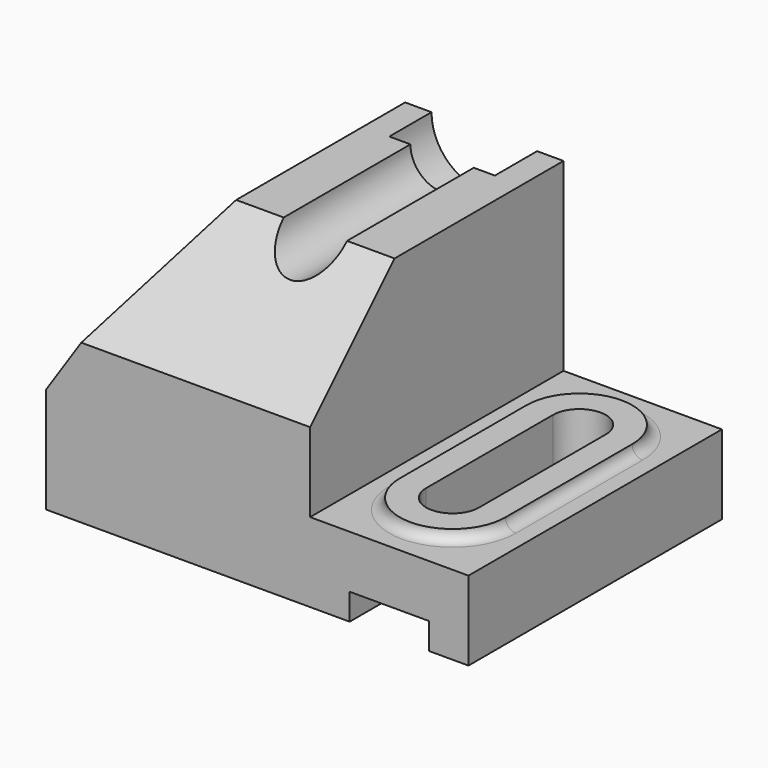
from build123d import *

# Parameters (mm, degrees)
F0_W         = 80
F0_H         = 60
F1_DEPTH     = 50
F2_W         = 30
F2_H         = 33
F3_DEPTH     = 60.001
F5_DEPTH     = 17.001
F6_W         = 30
F6_H         = 60
F7_DEPTH     = 2
F8_W         = 15
F8_H         = 5
F9_DEPTH     = 60.001
F10_R        = 1.99999
F12_DEPTH    = 60.001
F13_W        = 6
F13_H        = 48.9288835973
F15_W        = 4
F15_H        = 10
F17_T1_DEPTH = 132.8673195186


# Not quite as in the source:
# - a fillet or chamfer that OpenCascade refuses, or shapes differently, is made with other operations: its cross-section is extruded or revolved along the edge and cut away or added
# - a fillet or chamfer is up to 0.001 mm smaller than in the source, because OpenCascade refuses the exact size


with BuildPart() as f1:
    # F0 (on Top) → F1 (new body)
    with BuildSketch(Plane.XY):
        Rectangle(F0_W, F0_H)
    extrude(amount=F1_DEPTH)

    # F2 (on face) → F3 (cut, through all)
    with BuildSketch(Plane.XZ.offset(30)):
        with Locations((25, 33.5)):
            Rectangle(F2_W, F2_H)
    extrude(amount=-F3_DEPTH, mode=Mode.SUBTRACT)

    # F4 (on face) → F5 (cut, through all)
    with BuildSketch(Plane.XY.offset(17)):
        with BuildLine():
            ThreePointArc((20, -15), (25, -20), (30, -15))
            Line((30, -15), (30, 15))
            ThreePointArc((30, 15), (25, 20), (20, 15))
            Line((20, 15), (20, -15))
        make_face()
    extrude(amount=-F5_DEPTH, mode=Mode.SUBTRACT)

    # F6 (on face) → F7 (cut)
    with BuildSketch(Plane.XY.offset(17)):
        with Locations((25, 0)):
            Rectangle(F6_W, F6_H)
        with BuildLine():
            Line((35, 15), (35, -15))
            ThreePointArc((35, -15), (25, -25), (15, -15))
            Line((15, -15), (15, 15))
            ThreePointArc((15, 15), (25, 25), (35, 15))
        make_face(mode=Mode.SUBTRACT)
    extrude(amount=-F7_DEPTH, mode=Mode.SUBTRACT)

    # F8 (on face) → F9 (cut, through all)
    with BuildSketch(Plane.XZ.offset(30)):
        with Locations((25, 2.5)):
            Rectangle(F8_W, F8_H)
    extrude(amount=-F9_DEPTH, mode=Mode.SUBTRACT)

    # F10 (radius 2 in the source; OpenCascade refuses exactly that, so slightly less here)
    f10_edges = [f1.edges().sort_by_distance(p)[0] for p in [
        (35, 0, 15),
    ]]
    fillet(f10_edges, radius=F10_R)

    # F11 (on face) → F12 (cut, through all)
    with BuildSketch(Plane.XZ.offset(30)):
        Polygon((-40, 20), (-20, 50), (-40, 50), align=None)
    extrude(amount=-F12_DEPTH, mode=Mode.SUBTRACT)

    # F13 (on face) → F14 (revolve, cut)
    with BuildSketch(Plane.XY.offset(50)):
        with Locations((-8, 5.5355582014)):
            Rectangle(F13_W, F13_H)
    revolve(axis=Axis((-5, -1.603256911, 50), (0, -1, 0)), mode=Mode.SUBTRACT)

    # F15 (on face) → F16 (revolve, cut)
    with BuildSketch(Plane.XY.offset(50)):
        with Locations((-13, 25)):
            Rectangle(F15_W, F15_H)
    revolve(axis=Axis((-5, 25, 50), (0, -1, 0)), mode=Mode.SUBTRACT)

    # F17: chamfer of 20 on 1 edges, made by hand

    # F17_s2 → F17_t1 (cut)
    with BuildSketch(Plane.YZ.offset(-71.4336597593)):
        Polygon((-30, 30), (-10, 50), (-30, 50), align=None)
    extrude(amount=F17_T1_DEPTH, mode=Mode.SUBTRACT)


solid = f1.part
